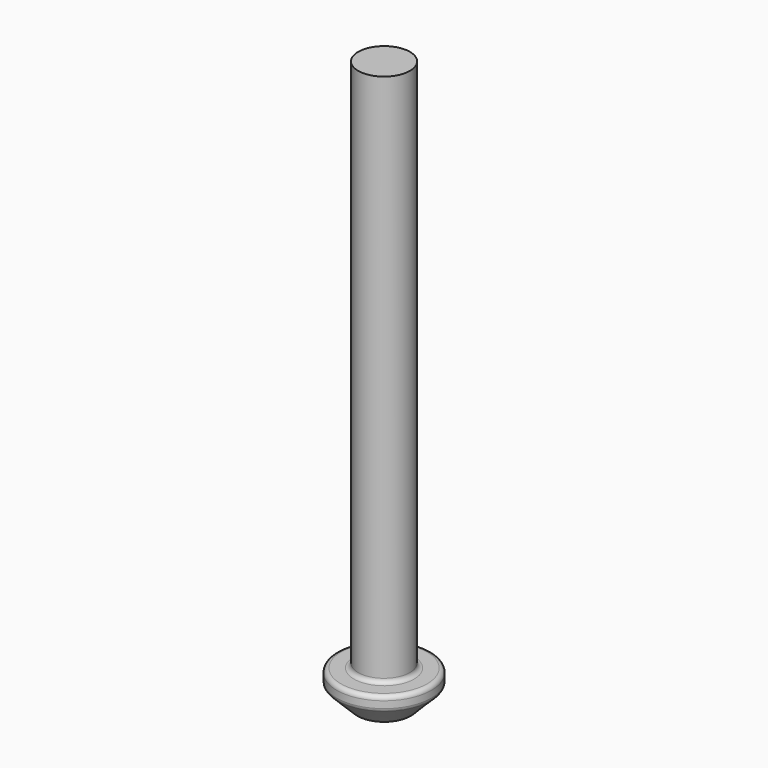
from build123d import *

# Parameters (mm, degrees)
F1_R     = 2.75
F1_R_2   = 1.5
F2_DEPTH = 2
F3_START = 1.5
F3_DEPTH = 0.5
F4_START = 2
F4_DEPTH = 31
F5_SIZE2 = 1.25
F5_SIZE  = 1.25
F6_R     = 0.25


# Not quite as in the source:
# - a feature names something its author has since deleted; it is built from what else it names


with BuildPart() as f2:
    # F1 (on Top) → F2 (new body)
    with BuildSketch(Plane.XY):
        Circle(F1_R)
        Circle(F1_R_2, mode=Mode.SUBTRACT)
        Circle(F1_R_2)
        Polygon((-0.5773502692, -1), (-1.1547005384, 0), (-0.5773502692, 1), (0.5773502692, 1), (1.1547005384, 0), (0.5773502692, -1), align=None, mode=Mode.SUBTRACT)
    extrude(amount=F2_DEPTH)

    # F1 (on Top) → F3 (join)
    with BuildSketch(Plane.XY.offset(F3_START)):
        Polygon((-0.5773502692, 1), (-1.1547005384, 0), (-0.5773502692, -1), (0.5773502692, -1), (1.1547005384, 0), (0.5773502692, 1), align=None)
    extrude(amount=F3_DEPTH)

    # F1 (on Top) → F4 (join)
    with BuildSketch(Plane.XY.offset(F4_START)):
        Circle(F1_R_2)
        Polygon((-0.5773502692, -1), (-1.1547005384, 0), (-0.5773502692, 1), (0.5773502692, 1), (1.1547005384, 0), (0.5773502692, -1), align=None, mode=Mode.SUBTRACT)
        Polygon((-0.5773502692, 1), (-1.1547005384, 0), (-0.5773502692, -1), (0.5773502692, -1), (1.1547005384, 0), (0.5773502692, 1), align=None)
    extrude(amount=F4_DEPTH)

    # F5
    f5_edges = [f2.edges().sort_by_distance(p)[0] for p in [
        (-2.75, 0, 0),
    ]]
    chamfer(f5_edges, length=F5_SIZE, length2=F5_SIZE2)

    # F6
    f6_edges = [f2.edges().sort_by_distance(p)[0] for p in [
        (-2.75, 0, 2),
        (-1.5, 0, 2),
        (-1.5, 0, 0),
        (-2.75, 0, 1.25),
    ]]
    fillet(f6_edges, radius=F6_R)


solid = f2.part
